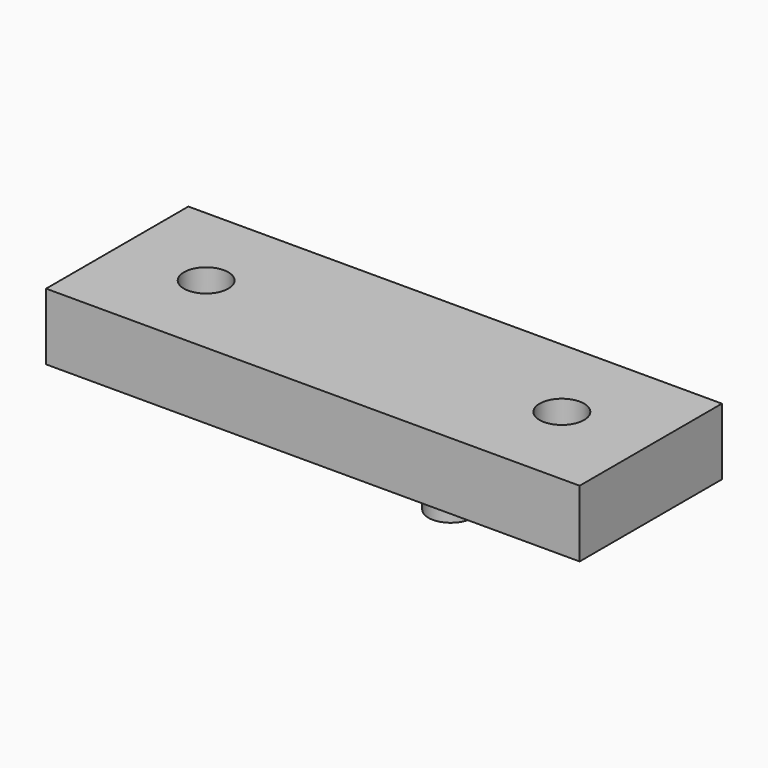
from build123d import *

# Parameters (mm, degrees)
F0_W          = 120
F0_H          = 40
F0_R          = 5
F1_DEPTH      = 15
F2_R          = 5
F3_DEPTH      = 2.5
F4_DEPTH      = 12.5
F4_DEPTH_BACK = 2.5
F5_DEPTH      = 2.5
F5_DEPTH_BACK = 12.5
F6_R          = 5
F7_DEPTH      = 5


with BuildPart() as f1:
    # F0 (on Top) → F1 (new body)
    with BuildSketch(Plane.XY):
        Rectangle(F0_W, F0_H)
        with Locations((-40, 0)):
            Circle(F0_R, mode=Mode.SUBTRACT)
        with Locations((40, 0)):
            Circle(F0_R, mode=Mode.SUBTRACT)
    extrude(amount=F1_DEPTH)


with BuildPart() as f3:
    # F2 (on Top) → F3 (new body, symmetric)
    with BuildSketch(Plane.XY):
        with BuildLine():
            ThreePointArc((15, -10), (25, 0), (15, 10))
            Line((15, 10), (-15, 10))
            ThreePointArc((-15, 10), (-25, 0), (-15, -10))
            Line((-15, -10), (15, -10))
        make_face()
        with Locations((-15, 0)):
            Circle(F2_R, mode=Mode.SUBTRACT)
        with Locations((15, 0)):
            Circle(F2_R, mode=Mode.SUBTRACT)
    extrude(amount=F3_DEPTH, both=True)

    # F2 (on Top) → F4 (join, two sides)
    with BuildSketch(Plane.XY) as f4_sk:
        with Locations((-15, 0)):
            Circle(F2_R)
    extrude(amount=F4_DEPTH)
    extrude(f4_sk.sketch, amount=-F4_DEPTH_BACK)

    # F2 (on Top) → F5 (join, two sides)
    with BuildSketch(Plane.XY) as f5_sk:
        with Locations((15, 0)):
            Circle(F2_R)
    extrude(amount=F5_DEPTH)
    extrude(f5_sk.sketch, amount=-F5_DEPTH_BACK)


with BuildPart() as f7:
    # F6 (on Top) → F7 (new body, symmetric)
    with BuildSketch(Plane.XY):
        with BuildLine():
            Line((-40, -10), (40, -10))
            ThreePointArc((40, -10), (50, 0), (40, 10))
            Line((40, 10), (-40, 10))
            ThreePointArc((-40, 10), (-50, 0), (-40, -10))
        make_face()
        with Locations((-40, 0)):
            Circle(F6_R, mode=Mode.SUBTRACT)
        with Locations((40, 0)):
            Circle(F6_R, mode=Mode.SUBTRACT)
    extrude(amount=F7_DEPTH, both=True)


solid = Compound([f1.part, f3.part, f7.part])
